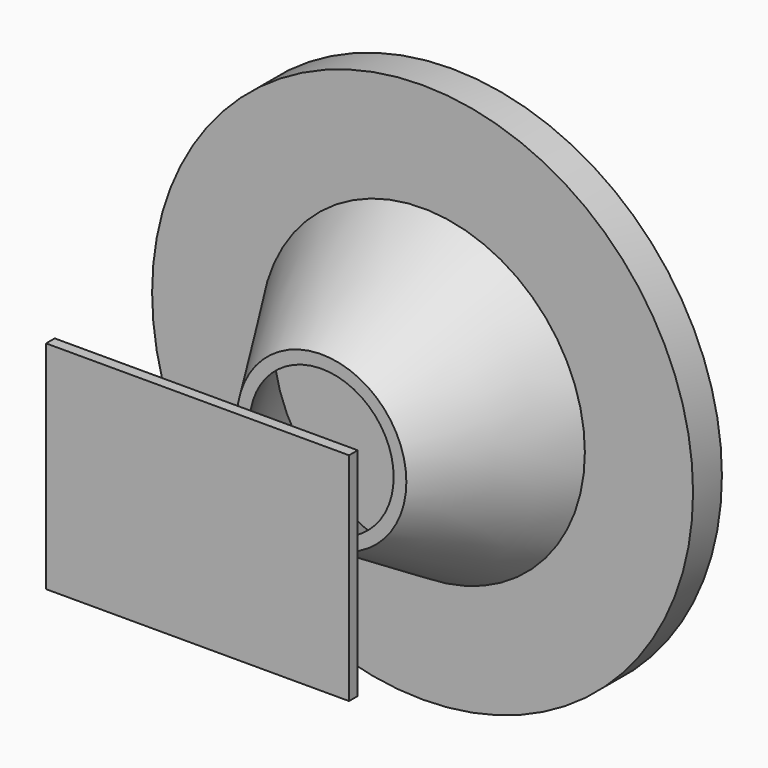
from build123d import *

# Parameters (mm, degrees)
F1_DEPTH = 30
F4_R     = 71.5
F5_DEPTH = 4


with BuildPart() as f1:
    # F0 (on Top) → F1 (new body, symmetric)
    with BuildSketch(Plane.XY):
        Polygon((0, -40), (-23.5, -40), (-42, -40), (-42, -43), (0, -43), align=None)
        Polygon((23.5, -40), (0, -40), (0, -43), (42, -43), (42, -40), align=None)
    extrude(amount=F1_DEPTH, both=True)


with BuildPart() as f2:
    # F0 (on Top) → F2 (revolve)
    with BuildSketch(Plane.XY):
        Polygon((41.479187246, 35), (19.979187246, 0), (23.5, 0), (45, 35), align=None)
    revolve(axis=Axis((0, 17.5, 0), (0, -1, 0)))


with BuildPart() as f3:
    # F0 (on Top) → F3 (revolve)
    with BuildSketch(Plane.XY):
        Polygon((-75, 35), (-45, 35), (0, 35), (0, 45), (-75, 45), align=None)
    revolve(axis=Axis((0, 40, 0), (0, -1, 0)))

    # F4 (on face) → F5 (cut, symmetric)
    with BuildSketch(Plane(origin=(0, 45, 0), x_dir=(-1, 0, 0), z_dir=(0, 1, 0))):
        with Locations((-0.5644535995, 0)):
            Circle(F4_R)
    extrude(amount=F5_DEPTH, both=True, mode=Mode.SUBTRACT)


solid = Compound([f1.part, f2.part, f3.part])
